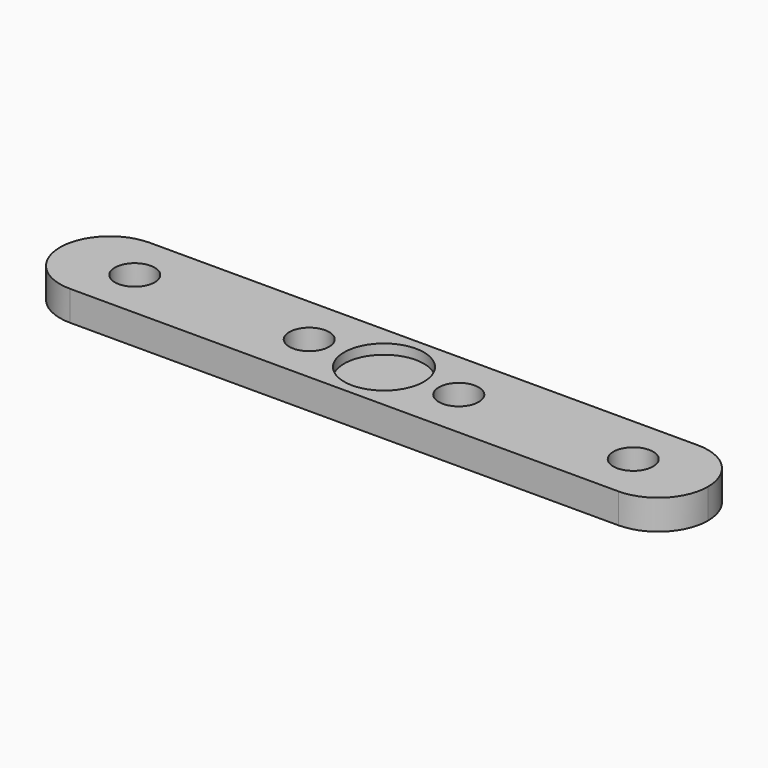
from build123d import *

# Parameters (mm, degrees)
F0_W     = 65
F0_H     = 10
F1_DEPTH = 3
F2_R     = 4
F3_DEPTH = 1
F4_R     = 2
F5_DEPTH = 25
F6_R     = 4.99999


# Not quite as in the source:
# - a fillet or chamfer is up to 0.001 mm smaller than in the source, because OpenCascade refuses the exact size


with BuildPart() as f1:
    # F0 (on Top) → F1 (new body)
    with BuildSketch(Plane.XY):
        Rectangle(F0_W, F0_H)
    extrude(amount=F1_DEPTH)

    # F2 (on face) → F3 (cut)
    with BuildSketch(Plane.XY.offset(3)):
        Circle(F2_R)
    extrude(amount=-F3_DEPTH, mode=Mode.SUBTRACT)

    # F4 (on face) → F5 (cut)
    with BuildSketch(Plane.XY.offset(3)):
        with Locations((-7.5, 0)):
            Circle(F4_R)
        with Locations((7.5, 0)):
            Circle(F4_R)
        with Locations((-25, 0)):
            Circle(F4_R)
        with Locations((25, 0)):
            Circle(F4_R)
    extrude(amount=-F5_DEPTH, mode=Mode.SUBTRACT)

    # F6 (radius 5 in the source; OpenCascade refuses exactly that, so slightly less here)
    f6_edges = [f1.edges().sort_by_distance(p)[0] for p in [
        (-32.5, -5, 1.5),
        (-32.5, 5, 1.5),
        (32.5, -5, 1.5),
        (32.5, 5, 1.5),
    ]]
    fillet(f6_edges, radius=F6_R)


solid = f1.part
